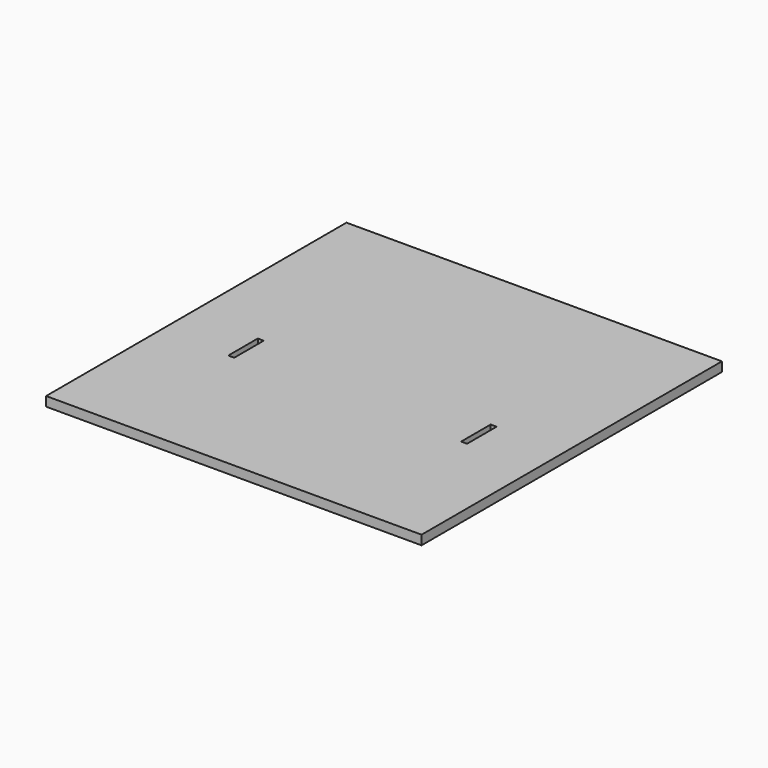
from build123d import *

# Parameters (mm, degrees)
F0_W     = 2.0066
F0_H     = 12.4968
F0_W_2   = 19.05
F0_H_2   = 12.7
F0_H_3   = 1.27
F1_DEPTH = 3.175


# Not quite as in the source:
# - a length typed as a fraction of an inch, garbled in the dataset ("3 / 203.2 mm" for 3/8 in), is restored


with BuildPart() as f1:
    # F0 (on Top) → F1 (new body)
    with BuildSketch(Plane.XY):
        Polygon((-63.5, 0), (0, 0), (0, 127), (-63.5, 127), (-63.5, 13.97), (-44.45, 13.97), (-44.45, 12.7), (-63.5, 12.7), align=None)
        with Locations((-24.1173, 54.3814)):
            Rectangle(F0_W, F0_H, mode=Mode.SUBTRACT)
        Polygon((-95.25, 0), (-82.55, 0), (-82.55, 12.7), (-82.55, 13.97), (-63.5, 13.97), (-63.5, 127), (-127, 127), (-127, 54.3814), (-127, 0), align=None)
        Polygon((-103.886, 48.133), (-103.886, 54.3814), (-103.886, 60.6298), (-101.8794, 60.6298), (-101.8794, 48.133), align=None, mode=Mode.SUBTRACT)
        with Locations((-73.025, 6.35)):
            Rectangle(F0_W_2, F0_H_2)
        with Locations((-73.025, 13.335)):
            Rectangle(F0_W_2, F0_H_3)
        with Locations((-53.975, 13.335)):
            Rectangle(F0_W_2, F0_H_3)
    extrude(amount=F1_DEPTH)


solid = f1.part
